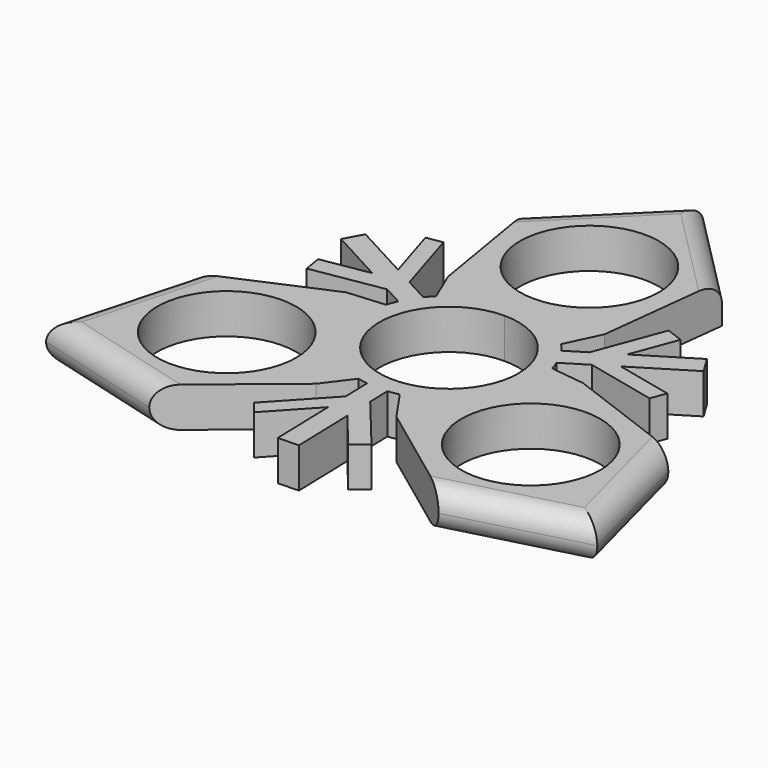
from build123d import *

# Parameters (mm, degrees)
F0_R     = 11.049
F1_DEPTH = 6.35
F2_R     = 3.17499


# Not quite as in the source:
# - a fillet or chamfer is up to 0.001 mm smaller than in the source, because OpenCascade refuses the exact size


with BuildPart() as f1:
    # F0 (on Top) → F1 (new body)
    with BuildSketch(Plane.XY):
        with BuildLine():
            ThreePointArc((10.266368543, 9.474311423), (5.6037830713, 12.7968166076), (0, 13.97))
            ThreePointArc((0, 13.97), (-5.3724040771, 12.8956649473), (-9.9185000629, 9.8378989882))
            ThreePointArc((-9.9185000629, 9.8378989882), (-10.4709665549, 9.247689409), (-10.9883672437, 8.6265106107))
            Line((-10.9883672437, 8.6265106107), (-14.8673558727, 10.7216511471))
            Line((-14.8673558727, 10.7216511471), (-18.2652639065, 21.743875915))
            Line((-18.2652639065, 21.743875915), (-20.7996486885, 21.3214784899))
            Line((-20.7996486885, 21.3214784899), (-18.0642706589, 12.4483862321))
            Line((-18.0642706589, 12.4483862321), (-27.1912532422, 17.3781019425))
            Line((-27.1912532422, 17.3781019425), (-28.7577700617, 14.4778187277))
            Line((-28.7577700617, 14.4778187277), (-19.9750544664, 9.7340503842))
            Line((-19.9750544664, 9.7340503842), (-27.5974388749, 8.4636530986))
            Line((-27.5974388749, 8.4636530986), (-27.1215043395, 5.6080456262))
            Line((-27.1215043395, 5.6080456262), (-15.8225889535, 7.4911980188))
            Line((-15.8225889535, 7.4911980188), (-12.7056009028, 5.8076333991))
            ThreePointArc((-12.7056009028, 5.8076333991), (-13.0481194381, 4.9907393369), (-13.3381786472, 4.1537802513))
            ThreePointArc((-13.3381786472, 4.1537802513), (-12.2222121685, -6.7659758874), (-3.5606204122, -13.508622516))
            ThreePointArc((-3.5606204122, -13.508622516), (-2.773250677, -13.6919677433), (-1.9765937131, -13.8294604845))
            Line((-1.9765937131, -13.8294604845), (-1.8515443275, -18.2363334465))
            Line((-1.8515443275, -18.2363334465), (-9.6981169659, -26.6901205073))
            Line((-9.6981169659, -26.6901205073), (-8.0651176742, -28.6737633989))
            Line((-8.0651176742, -28.6737633989), (-1.7484833836, -21.8683104075))
            Line((-1.7484833836, -21.8683104075), (-1.4542511306, -32.2373670397))
            Line((-1.4542511306, -32.2373670397), (1.8407262213, -32.1438687935))
            Line((1.8407262213, -32.1438687935), (1.5575923187, -22.165929802))
            Line((1.5575923187, -22.165929802), (6.4689808452, -28.1319096943))
            Line((6.4689808452, -28.1319096943), (8.7040421919, -26.29193456))
            Line((8.7040421919, -26.29193456), (1.4237266877, -17.4483629968))
            Line((1.4237266877, -17.4483629968), (1.323242392, -13.9071898517))
            ThreePointArc((1.323242392, -13.9071898517), (2.2019526696, -13.7953725735), (3.0718101042, -13.6280916743))
            ThreePointArc((3.0718101042, -13.6280916743), (11.9706130841, -7.2017582846), (13.4791204751, 3.6707235278))
            ThreePointArc((13.4791204751, 3.6707235278), (13.244217232, 4.4442783342), (12.9649609568, 5.2029498738))
            Line((12.9649609568, 5.2029498738), (16.7189002003, 7.5146822993))
            Line((16.7189002003, 7.5146822993), (27.9633808724, 4.9462445923))
            Line((27.9633808724, 4.9462445923), (28.8647663627, 7.3522849091))
            Line((28.8647663627, 7.3522849091), (19.8127540426, 9.4199241754))
            Line((19.8127540426, 9.4199241754), (28.6455043728, 14.8592650972))
            Line((28.6455043728, 14.8592650972), (26.9170438404, 17.6660500658))
            Line((26.9170438404, 17.6660500658), (18.9289850868, 12.7468829615))
            Line((18.9289850868, 12.7468829615), (18.4174621476, 12.4318794178))
            Line((18.4174621476, 12.4318794178), (21.1284580297, 19.6682565957))
            Line((21.1284580297, 19.6682565957), (18.4174621476, 20.6838889338))
            Line((18.4174621476, 20.6838889338), (14.3988622659, 9.957164978))
            Line((14.3988622659, 9.957164978), (11.3823585109, 8.0995564527))
            ThreePointArc((11.3823585109, 8.0995564527), (10.8461667685, 8.8046332365), (10.266368543, 9.474311423))
        make_face()
        with BuildLine():
            ThreePointArc((0, 11.049), (7.8128228253, 7.8128228253), (11.049, 0))
            ThreePointArc((11.049, 0), (-7.8128228253, -7.8128228253), (0, 11.049))
        make_face(mode=Mode.SUBTRACT)
        with BuildLine():
            ThreePointArc((-9.9185000629, 9.8378989882), (-5.3724040771, 12.8956649473), (0, 13.97))
            ThreePointArc((0, 13.97), (5.6037830713, 12.7968166076), (10.266368543, 9.474311423))
            Line((10.266368543, 9.474311423), (12.8332442979, 14.8954782635))
            Line((12.8332442979, 14.8954782635), (15.1805052923, 35.3235639632))
            Line((15.1805052923, 35.3235639632), (0, 50.6446287036))
            Line((0, 50.6446287036), (-15.4629256576, 35.3235639632))
            Line((-15.4629256576, 35.3235639632), (-12.0582450181, 14.8954782635))
            Line((-12.0582450181, 14.8954782635), (-9.9185000629, 9.8378989882))
        make_face()
        with BuildLine():
            ThreePointArc((11.049, 27.94), (7.8128228253, 20.1271771747), (0, 16.891))
            ThreePointArc((0, 16.891), (-7.8128228253, 35.7528228253), (11.049, 27.94))
        make_face(mode=Mode.SUBTRACT)
        with BuildLine():
            ThreePointArc((-3.5606204122, -13.508622516), (-12.2222121685, -6.7659758874), (-13.3381786472, 4.1537802513))
            Line((-13.3381786472, 4.1537802513), (-19.3164847266, 3.6661764432))
            Line((-19.3164847266, 3.6661764432), (-38.1813563905, -4.5150787562))
            Line((-38.1813563905, -4.5150787562), (-43.8595350225, -25.3223143518))
            Line((-43.8595350225, -25.3223143518), (-22.8596409155, -31.0530684179))
            Line((-22.8596409155, -31.0530684179), (-6.8707400686, -17.8904856425))
            Line((-6.8707400686, -17.8904856425), (-3.5606204122, -13.508622516))
        make_face()
        with Locations((-24.1967497817, -13.97)):
            Circle(F0_R, mode=Mode.SUBTRACT)
        with BuildLine():
            Line((18.9289850868, 2.995007379), (13.4791204751, 3.6707235278))
            ThreePointArc((13.4791204751, 3.6707235278), (11.9706130841, -7.2017582846), (3.0718101042, -13.6280916743))
            Line((3.0718101042, -13.6280916743), (6.4832404288, -18.5616547067))
            Line((6.4832404288, -18.5616547067), (23.0008510982, -30.808485207))
            Line((23.0008510982, -30.808485207), (43.8595350225, -25.3223143518))
            Line((43.8595350225, -25.3223143518), (38.3225665731, -4.2704955452))
            Line((38.3225665731, -4.2704955452), (18.9289850868, 2.995007379))
        make_face()
        with Locations((24.1967497817, -13.97)):
            Circle(F0_R, mode=Mode.SUBTRACT)
    extrude(amount=F1_DEPTH)

    # F2 (radius 3.175 in the source; OpenCascade refuses exactly that, so slightly less here)
    f2_edges = [f1.edges().sort_by_distance(p)[0] for p in [
        (-7.731463, 42.984096, 6.35),
        (7.590253, 42.984096, 6.35),
        (41.091051, -14.796405, 6.35),
        (33.430193, -28.0654, 6.35),
        (-41.020446, -14.918697, 6.35),
        (-33.359588, -28.187691, 6.35),
        (-33.359588, -28.187691, 0),
        (-41.020446, -14.918697, 0),
        (-7.731463, 42.984096, 0),
        (41.091051, -14.796405, 0),
        (33.430193, -28.0654, 0),
    ]]
    fillet(f2_edges, radius=F2_R)


solid = f1.part
